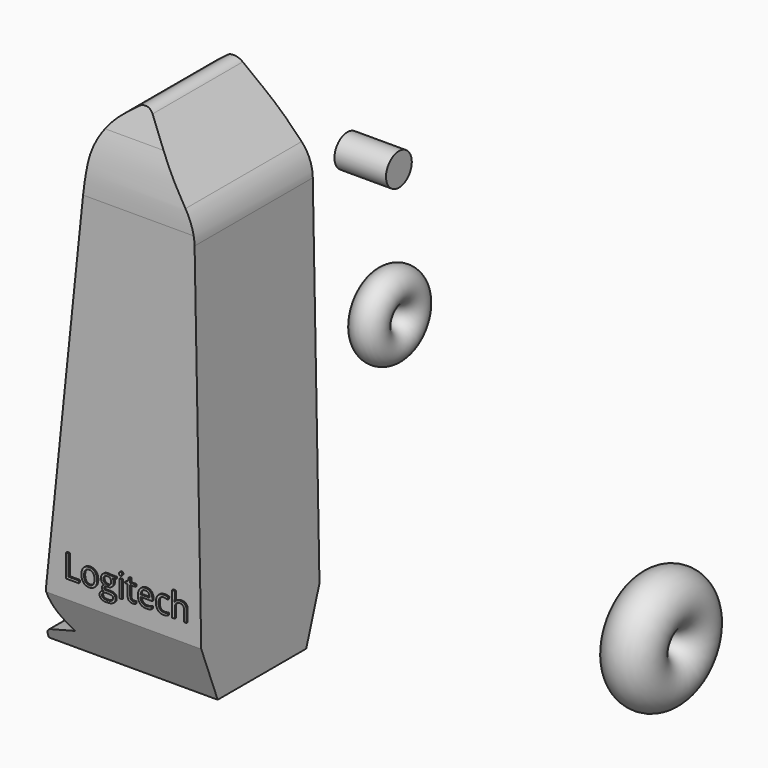
from build123d import *

# Parameters (mm, degrees)
F1_DEPTH      = 21.844
F2_R          = 14.7055024853
F3_R          = 3.0383878795
F4_R          = 20.0456056877
F5_R          = 11.8075289687
F6_R          = 2.1063902844
F8_DEPTH      = 45.974
F9_R          = 61.4792288787
F10_R         = 52.1493472686
F11_TEXT_SIZE = 9.5077221178
F12_DEPTH     = 22.2758
F13_R         = 4.8631269679
F13_R_2       = 7.768423192
F16_R         = 4.7665861038
F17_DEPTH     = 15.24


# Not quite as in the source:
# - Text() gives the source's letters only with a copy of the font that has no kerning and outlines rounded to 1/6400 em; it was checked with that copy


with BuildPart() as f1:
    # F0 (on Front) → F1 (new body, symmetric)
    with BuildSketch(Plane.XZ):
        Polygon((18.5026712716, 48.6062318087), (0, 72.9827731848), (-12.6288104802, 63.2908865809), (-25.8450061083, -64.1719698906), (-19.6774490178, -70.3395232558), (-29.0756318718, -73.2764601707), (-29.0756318718, -75.9197026491), (20.8522174507, -75.9197026491), align=None)
    extrude(amount=F1_DEPTH, both=True)

    # F2
    f2_edges = [f1.edges().sort_by_distance(p)[0] for p in [
        (18.502671, 0, 48.606232),
    ]]
    fillet(f2_edges, radius=F2_R)

    # F3
    f3_edges = [f1.edges().sort_by_distance(p)[0] for p in [
        (0, 0, 72.982773),
    ]]
    fillet(f3_edges, radius=F3_R)

    # F4
    f4_edges = [f1.edges().sort_by_distance(p)[0] for p in [
        (-12.62881, 0, 63.290887),
    ]]
    fillet(f4_edges, radius=F4_R)

    # F5
    f5_edges = [f1.edges().sort_by_distance(p)[0] for p in [
        (-25.845006, 0, -64.17197),
    ]]
    fillet(f5_edges, radius=F5_R)

    # F6
    f6_edges = [f1.edges().sort_by_distance(p)[0] for p in [
        (-29.075632, 0, -73.27646),
    ]]
    fillet(f6_edges, radius=F6_R)

    # F7 (on Right) → F8 (cut, symmetric)
    with BuildSketch(Plane.YZ):
        Polygon((16.3798201829, 72.1387192607), (22.0600292087, 54.604165256), (22.0600292087, 72.1387192607), align=None)
        Polygon((-22.524273023, 72.1387192607), (-22.0876950771, 54.604165256), (-15.8882923424, 72.1387192607), align=None)
        Polygon((-15.8882923424, -76.5606984496), (-22.524273023, -58.6556904018), (-22.524273023, -76.5606984496), align=None)
        Polygon((22.7101982368, -58.6556904018), (16.3798201829, -76.5606984496), (22.7101982368, -76.5606984496), align=None)
    extrude(amount=F8_DEPTH, both=True, mode=Mode.SUBTRACT)

    # F9
    f9_edges = [f1.edges().sort_by_distance(p)[0] for p in [
        (-0.004241, 21.844, 55.271038),
    ]]
    fillet(f9_edges, radius=F9_R)

    # F10
    f10_edges = [f1.edges().sort_by_distance(p)[0] for p in [
        (-0.011254, -21.844, 55.293439),
    ]]
    fillet(f10_edges, radius=F10_R)

    # F11 (on Front) → F12 (join)
    with BuildSketch(Plane.XZ):
        with Locations((-20.0259014964, -54.8532344401)):
            Text('Logitech', F11_TEXT_SIZE, font='Open Sans', text_align=(TextAlign.LEFT, TextAlign.BOTTOM))
    extrude(amount=F12_DEPTH)


with BuildPart() as f14:
    # F13 (on Front) → F14 (revolve)
    with BuildSketch(Plane.XZ):
        with Locations((58.8279701769, 37.6955904067)):
            Circle(F13_R)
    revolve(axis=Axis((58.6861297488, 0, 30.121549964), (-1, 0, 0)))


with BuildPart() as f15:
    # F13 (on Front) → F15 (revolve)
    with BuildSketch(Plane.XZ):
        with Locations((139.0738934278, -17.9910790175)):
            Circle(F13_R_2)
    revolve(axis=Axis((139.0959471464, 0, -28.0732344836), (-1, 0, 0)))


with BuildPart() as f17:
    # F16 (on Right) → F17 (new body)
    with BuildSketch(Plane.YZ):
        with Locations((57.8730255365, 30.2572660148)):
            Circle(F16_R)
    extrude(amount=F17_DEPTH)


solid = Compound([f1.part, f14.part, f15.part, f17.part])
